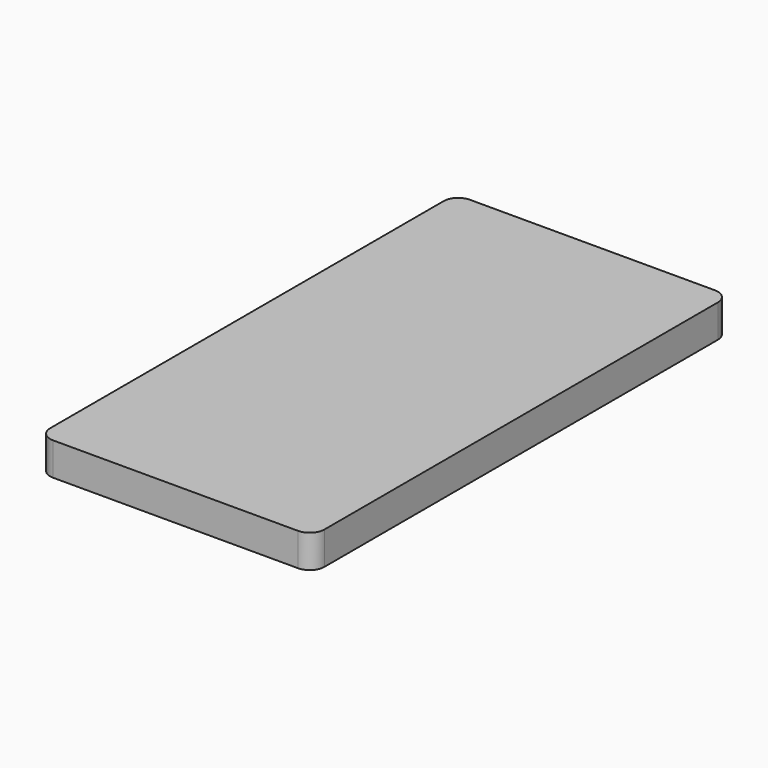
from build123d import *

# Parameters (mm, degrees)
F0_W     = 95.25
F0_H     = 180.975
F1_DEPTH = 11.43
F2_R     = 5.08


with BuildPart() as f1:
    # F0 (on Top) → F1 (new body)
    with BuildSketch(Plane.XY):
        with Locations((47.625, 90.4875)):
            Rectangle(F0_W, F0_H)
    extrude(amount=F1_DEPTH)

    # F2
    f2_edges = [f1.edges().sort_by_distance(p)[0] for p in [
        (0, 0, 5.715),
        (95.25, 0, 5.715),
        (0, 180.975, 5.715),
        (95.25, 180.975, 5.715),
    ]]
    fillet(f2_edges, radius=F2_R)


solid = f1.part
